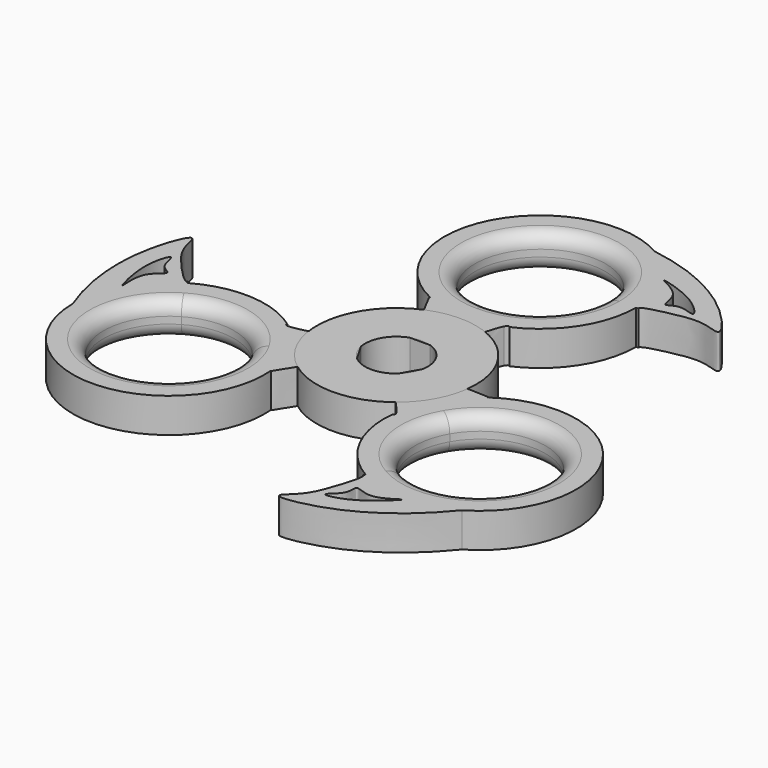
from build123d import *

# Parameters (mm, degrees)
F0_R     = 14.6321253096
F0_R_2   = 5.75
F2_DEPTH = 6.35
F3_R     = 2.54
F4_R     = 2.54
F5_COUNT = 3


# Not quite as in the source:
# - a feature names something its author has since deleted; it is built from what else it names


with BuildPart() as f2:
    # F0 (on Top) → F2 (new body)
    with BuildSketch(Plane.XY):
        Circle(F0_R)
        Circle(F0_R_2, mode=Mode.SUBTRACT)
    extrude(amount=-F2_DEPTH)


with BuildPart() as f2b:
    # F1 (on Top) → F2, piece 2 (new body)
    with BuildSketch(Plane.XY):
        with BuildLine():
            Line((0, 5.4448871638), (0, 15.3963098538))
            ThreePointArc((0, 15.3963098538), (-3.8147986955, 15.8138785868), (-7.4489333507, 17.0468092588))
            Line((-7.4489333507, 17.0468092588), (-7.4011550034, 16.8853468206))
            add(Edge.make_bspline(
                [(-4.5416971182, 11.304189338), (-4.9464033737, 12.1122090905), (-5.9307031021, 14.0443888842), (-7.6263386445, 16.8325787456), (-7.5310861985, 17.0853525935), (-7.4011550034, 16.8853468206)],
                knots=[0.0972300064, 0.0972300064, 0.0972300064, 0.0972300064, 0.4654294549, 0.9073619675, 1, 1, 1, 1], degree=3))
            ThreePointArc((-4.5416971182, 11.304189338), (-4.308050756, 10.6606233031), (-4.2287501997, 9.9805650074))
            Line((-4.2287501997, 9.9805650074), (-4.2287501997, 5.4448871638))
            Line((-4.2287501997, 5.4448871638), (0, 5.4448871638))
        make_face()
        with BuildLine():
            add(Edge.make_bspline(
                [(4.4865167549, 11.2358277593), (4.8136752679, 11.9669791972), (5.6531016297, 14.0180487359), (6.0143955866, 15.6492791849), (6.4483357613, 16.5476533946), (6.4971601168, 16.6368484914)],
                knots=[0.08910345, 0.08910345, 0.08910345, 0.08910345, 0.406197677, 0.7758100907, 0.8201313125, 0.8201313125, 0.8201313125, 0.8201313125], degree=3))
            ThreePointArc((6.4971601168, 16.6368484914), (3.307265702, 15.7092207304), (0, 15.3963098538))
            Line((0, 15.3963098538), (0, 5.4448871638))
            Line((0, 5.4448871638), (4.2287501997, 5.4448871638))
            Line((4.2287501997, 5.4448871638), (4.2287501997, 10.0286463653))
            ThreePointArc((4.2287501997, 10.0286463653), (4.2939100943, 10.6458437638), (4.4865167549, 11.2358277593))
        make_face()
        with BuildLine():
            add(Edge.make_bspline(
                [(6.4971601168, 16.6368484914), (6.6953038596, 16.9988286982), (6.9323322254, 17.2455739354), (7.190291953, 16.9288026722)],
                knots=[0.8201313125, 0.8201313125, 0.8201313125, 0.8201313125, 1, 1, 1, 1], degree=3))
            ThreePointArc((7.190291953, 16.9288026722), (14.7824433038, 23.4156382853), (17.6342287592, 32.9857541738))
            ThreePointArc((17.6342287592, 32.9857541738), (17.6342715188, 33.0081748817), (17.634285772, 33.0305956258))
            ThreePointArc((17.634285772, 33.0305956258), (15.2640329478, 41.8610731246), (8.7904534938, 48.3177131455))
            ThreePointArc((8.7904534938, 48.3177131455), (-15.6498331156, 41.1577573777), (-7.4489333507, 17.0468092588))
            ThreePointArc((-7.4489333507, 17.0468092588), (-3.8147986955, 15.8138785868), (0, 15.3963098538))
            ThreePointArc((0, 15.3963098538), (3.307265702, 15.7092207304), (6.4971601168, 16.6368484914))
        make_face()
        with BuildLine():
            ThreePointArc((12, 33.0305956258), (8.4852813742, 24.5453142515), (0, 21.0305956258))
            ThreePointArc((0, 21.0305956258), (-8.4852813742, 41.515877), (12, 33.0305956258))
        make_face(mode=Mode.SUBTRACT)
        with BuildLine():
            ThreePointArc((17.634285772, 33.0305956258), (17.6342715188, 33.0081748817), (17.6342287592, 32.9857541738))
            Line((17.6342287592, 32.9857541738), (18.0639845058, 32.9857541738))
            add(Edge.make_bspline(
                [(8.7904534938, 48.3177131455), (15.6092997036, 47.2735132728), (25.872444798, 42.7716458746), (33.5036552803, 33.1758988068), (28.1152865906, 35.5885745279), (23.5621846146, 34.941072322), (17.7328095973, 33.5470301335), (18.0639845058, 32.9857541738)],
                knots=[0.0351632128, 0.0351632128, 0.0351632128, 0.0351632128, 0.3009407692, 0.4872171144, 0.5969189571, 0.7557943985, 0.8995184196, 0.8995184196, 0.8995184196, 0.8995184196], degree=3))
            ThreePointArc((8.7904534938, 48.3177131455), (15.2640329478, 41.8610731246), (17.634285772, 33.0305956258))
        make_face()
        with BuildLine():
            add(Edge.make_bspline(
                [(15.4861349986, 42.115416912), (15.5210892778, 41.9542170992), (20.3147885724, 40.2088058164), (19.7584567513, 35.2581031235), (22.2267946753, 37.8182086751), (26.6698223315, 35.4009490714), (22.4371069035, 40.5179893989), (15.4426224528, 42.316085168), (15.4861349986, 42.115416912)],
                knots=[0, 0, 0, 0, 0.1784147321, 0.3334944411, 0.4560658064, 0.5992558922, 0.7779018937, 1, 1, 1, 1], degree=3))
        make_face(mode=Mode.SUBTRACT)
    extrude(amount=-F2_DEPTH)

    # F3
    f3_edges = [f2b.edges().sort_by_distance(p)[0] for p in [
        (0, 45.030596, 0),
    ]]
    fillet(f3_edges, radius=F3_R)

    # F4
    f4_edges = [f2b.edges().sort_by_distance(p)[0] for p in [
        (0, 45.030596, -6.35),
    ]]
    fillet(f4_edges, radius=F4_R)


with BuildPart() as f5_1:
    # F5: instance of F2b
    add(f2b.part.rotate(Axis((0, 0, 0), (0, 0, 1)), 1 * 360 / F5_COUNT))


with BuildPart() as f5_2:
    # F5: instance of F2b
    add(f2b.part.rotate(Axis((0, 0, 0), (0, 0, 1)), 2 * 360 / F5_COUNT))


with BuildPart() as f5_3:
    # F5: instance of F2
    add(f2.part.rotate(Axis((0, 0, 0), (0, 0, 1)), 1 * 360 / F5_COUNT))


with BuildPart() as f5_4:
    # F5: instance of F2
    add(f2.part.rotate(Axis((0, 0, 0), (0, 0, 1)), 2 * 360 / F5_COUNT))


solid = Compound([f2.part, f2b.part, f5_1.part, f5_2.part, f5_3.part, f5_4.part])
